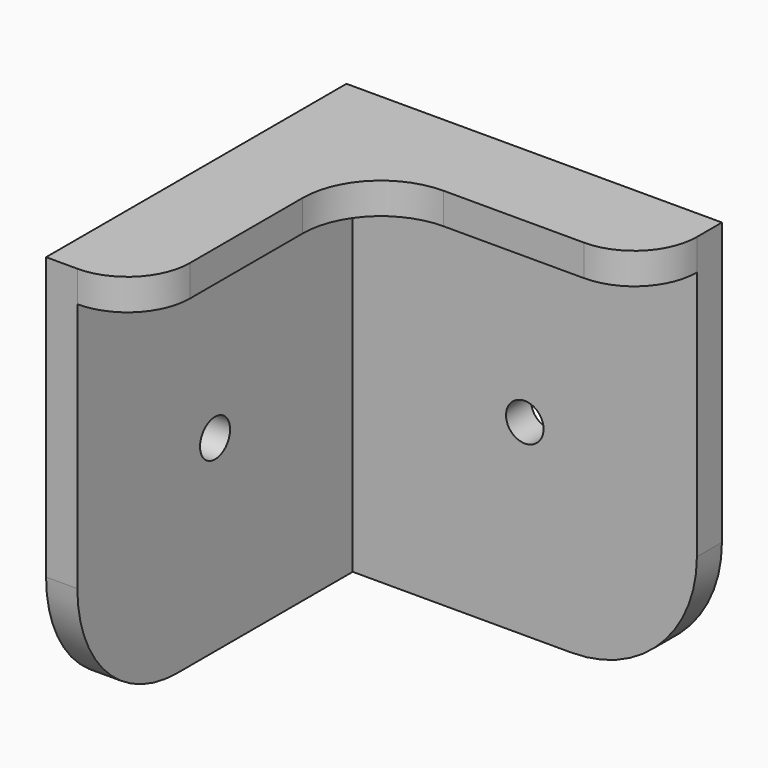
from build123d import *

# Parameters (mm, degrees)
F1_DEPTH  = 38.1
F3_DEPTH  = 3.175
F4_R      = 7.9375
F5_R      = 6.35
F9_R      = 12.7
F10_R     = 1.905
F11_DEPTH = 3.176


# Not quite as in the source:
# - a pattern or mirror of a feature is missing from the dataset's text; its kind, count and spacing are read off the source's solid


with BuildPart() as f1:
    # F0 (on Top) → F1 (new body)
    with BuildSketch(Plane.XY):
        Polygon((0, -34.925), (0, 0), (34.925, 0), (34.925, 3.175), (-3.175, 3.175), (-3.175, -34.925), align=None)
    extrude(amount=-F1_DEPTH)

    # F2 (on face) → F3 (join)
    with BuildSketch(Plane.XY):
        Polygon((6.35, -34.925), (6.35, -6.35), (34.925, -6.35), (34.925, 3.175), (-3.175, 3.175), (-3.175, -34.925), align=None)
    extrude(amount=F3_DEPTH)

    # F4
    f4_edges = [f1.edges().sort_by_distance(p)[0] for p in [
        (6.35, -6.35, 1.5875),
    ]]
    fillet(f4_edges, radius=F4_R)

    # F5
    f5_edges = [f1.edges().sort_by_distance(p)[0] for p in [
        (6.35, -34.925, 1.5875),
        (34.925, -6.35, 1.5875),
    ]]
    fillet(f5_edges, radius=F5_R)

    # F9
    f9_edges = [f1.edges().sort_by_distance(p)[0] for p in [
        (34.925, 1.5875, -38.1),
        (-1.5875, -34.925, -38.1),
    ]]
    fillet(f9_edges, radius=F9_R)

    # F10 (on face) → F11 (cut, through all)
    with BuildSketch(Plane.XZ):
        with Locations((17.4625, -19.05)):
            Circle(F10_R)
    f11 = extrude(amount=-F11_DEPTH, mode=Mode.SUBTRACT)

    # F11_copies: F11 across plane
    add(f11.mirror(Plane(origin=(0, 0, 0), x_dir=(0.7071067812, -0.7071067812, 0), z_dir=(-0.7071067812, -0.7071067812, 0))), mode=Mode.SUBTRACT)


solid = f1.part
